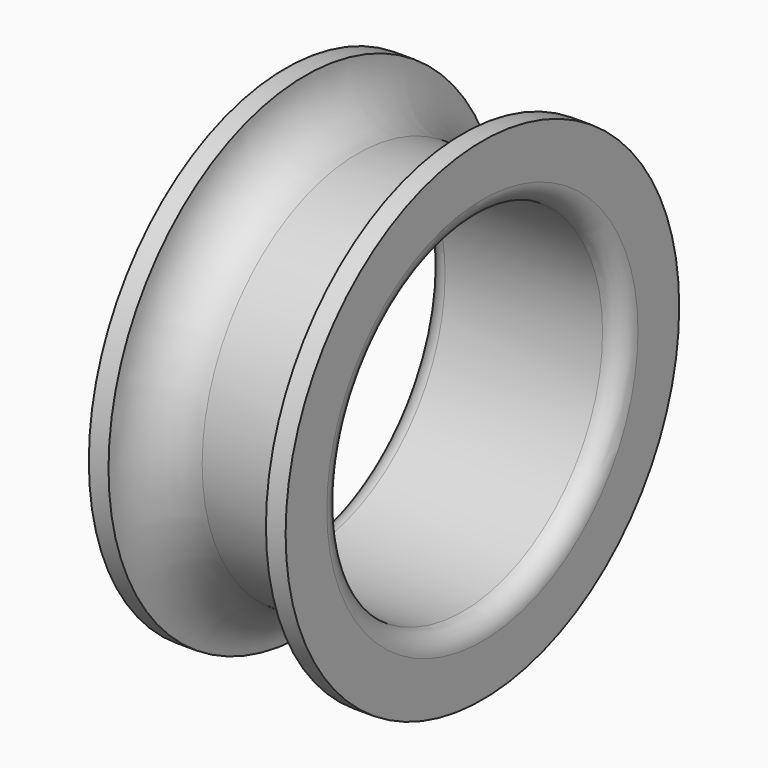
from build123d import *

# Parameters (mm, degrees)
F3_R = 3
F4_R = 1


# Not quite as in the source:
# - a fillet or chamfer that OpenCascade refuses, or shapes differently, is made with other operations: its cross-section is extruded or revolved along the edge and cut away or added


with BuildPart() as f1:
    # F0 (on Top) → F1 (revolve)
    with BuildSketch(Plane.XY):
        Polygon((-30, 26.65), (0, 26.65), (0, 37.5), (-3, 37.5), (-3, 29.65), (-27, 29.65), (-27, 37.5), (-30, 37.5), align=None)
    revolve(axis=Axis((5.0713585872, 0, 0), (1, 0, 0)))

    # F2: fillet of radius 8 on 1 edges, made by hand

    # F2_s1 → F2_t2 (revolve)
    with BuildSketch(Plane.XY):
        with BuildLine():
            ThreePointArc((-19.0014063736, 29.65), (-24.6049766641, 31.9403590306), (-27, 37.5))
            Line((-27, 37.5), (-27, 29.65))
            Line((-27, 29.65), (-19.0014063736, 29.65))
        make_face()
    revolve(axis=Axis((-27, 0, 0), (1, 0, 0)))

    # F3
    f3_edges = [f1.edges().sort_by_distance(p)[0] for p in [
        (0, -26.65, 0),
        (-30, -26.65, 0),
    ]]
    fillet(f3_edges, radius=F3_R)

    # F4
    f4_edges = [f1.edges().sort_by_distance(p)[0] for p in [
        (-3, -29.65, 0),
    ]]
    fillet(f4_edges, radius=F4_R)


solid = f1.part
